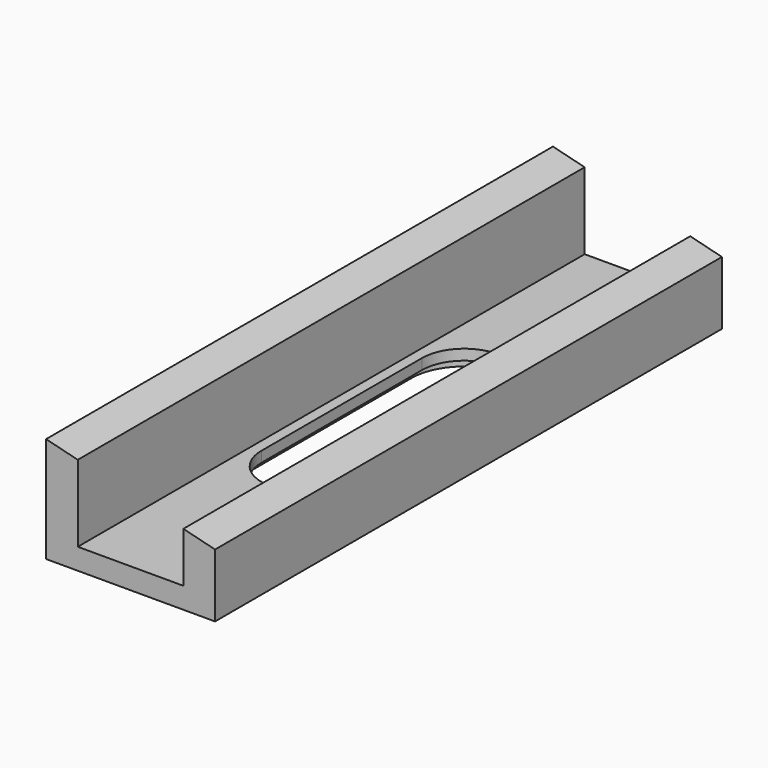
from build123d import *

# Parameters (mm, degrees)
F1_DEPTH = 60
F3_DEPTH = 2.001
F5_DEPTH = 1
F6_W     = 0.8
F6_H     = 3
F7_DEPTH = 1


# Not quite as in the source:
# - a feature names something its author has since deleted; it is built from what else it names


with BuildPart() as f1:
    # F0 (on Front) → F1 (new body)
    with BuildSketch(Plane.XZ):
        Polygon((0, 10), (0, 0), (16, 0), (16, 6), (13, 6.75), (13, 2), (3, 2), (3, 9.25), align=None)
    extrude(amount=F1_DEPTH)

    # F2 (on face) → F3 (cut, through all)
    with BuildSketch(Plane.XY.offset(2)):
        with BuildLine():
            ThreePointArc((12, -20.5), (8, -16.5), (4, -20.5))
            Line((4, -20.5), (4, -39.5))
            ThreePointArc((4, -39.5), (8, -43.5), (12, -39.5))
            Line((12, -39.5), (12, -20.5))
        make_face()
    extrude(amount=-F3_DEPTH, mode=Mode.SUBTRACT)

    # F4 (on Top) → F5 (cut)
    with BuildSketch(Plane.XY):
        with BuildLine():
            ThreePointArc((13, -20.5), (8, -15.5), (3, -20.5))
            Line((3, -20.5), (3, -39.5))
            ThreePointArc((3, -39.5), (8, -44.5), (13, -39.5))
            Line((13, -39.5), (13, -20.5))
        make_face()
    extrude(amount=F5_DEPTH, mode=Mode.SUBTRACT)

    # F6 (on Top) → F7 (join)
    with BuildSketch(Plane.XY):
        with Locations((6.8, -4.5)):
            Rectangle(F6_W, F6_H)
        with Locations((6.8, -55.5)):
            Rectangle(F6_W, F6_H)
    extrude(amount=-F7_DEPTH)


solid = f1.part
